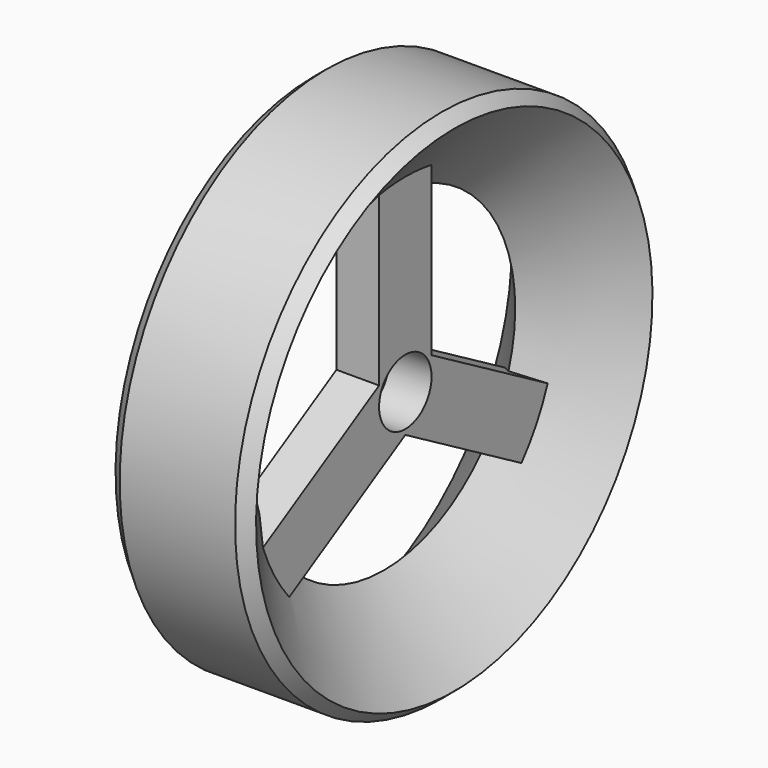
from build123d import *

# Parameters (mm, degrees)
F2_W            = 25.4
F2_H            = 73.3788463006
F3_DEPTH        = 8.255
F3_COPIES_COUNT = 3
F4_R            = 12.7
F5_DEPTH        = 35.4581824645


# Not quite as in the source:
# - a pattern or mirror of a feature is missing from the dataset's text; its kind, count and spacing are read off the source's solid


with BuildPart() as f1:
    # F0 (on Front) → F1 (revolve)
    with BuildSketch(Plane.XZ):
        Polygon((0, 73.3788463006), (-22.3378002507, 100), (-27.2021824645, 95.9182986785), (0, 63.5), (27.2021824645, 95.9182986785), (22.3378002507, 100), align=None)
    revolve(axis=Axis((12.7538797489, 0, 0), (1, 0, 0)))

    # F2 (on Right) → F3 (join, symmetric)
    with BuildSketch(Plane.YZ):
        with Locations((0, 36.6894231503)):
            Rectangle(F2_W, F2_H)
    f3 = extrude(amount=F3_DEPTH, both=True)

    # F3_copies: F3 ×3 about axis
    f3_copies_axis = Axis((0, 0, 0), (1, 0, 0))
    for i in range(1, F3_COPIES_COUNT):
        add(f3.rotate(f3_copies_axis, i * 360 / F3_COPIES_COUNT))

    # F4 (on face) → F5 (cut, through all)
    with BuildSketch(Plane(origin=(-8.255, 0, 0), x_dir=(0, -1, 0), z_dir=(-1, 0, 0))):
        Circle(F4_R)
    extrude(amount=-F5_DEPTH, mode=Mode.SUBTRACT)


with BuildPart() as f7:
    # F6 (on Front) → F7 (revolve)
    with BuildSketch(Plane.XZ):
        Polygon((22.3378002507, 100), (-22.3378002507, 100), (0, 73.3788463006), align=None)
    revolve(axis=Axis((4.5150928199, 0, 0), (1, 0, 0)))


solid = Compound([f1.part, f7.part])
